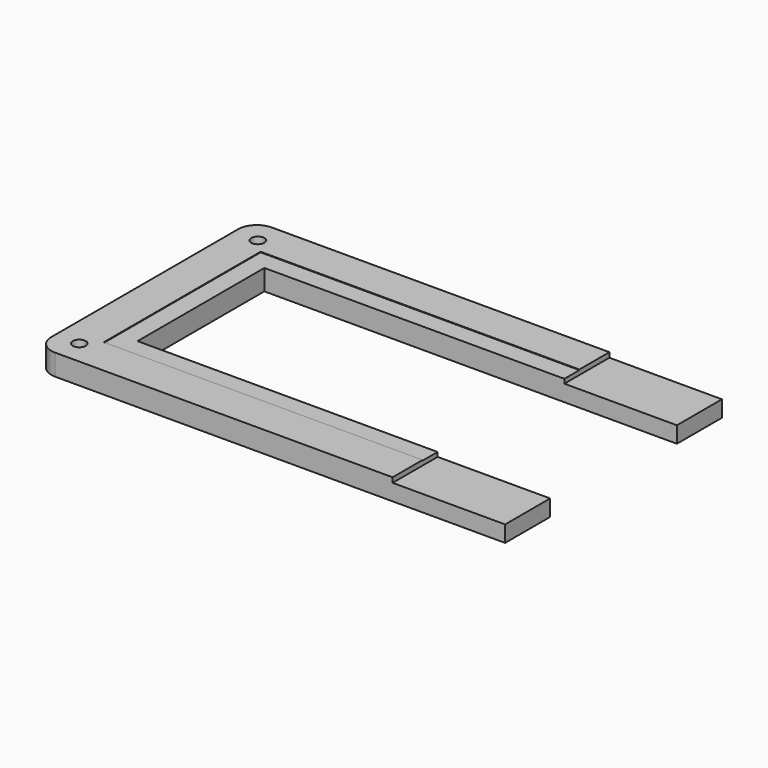
from build123d import *

# Parameters (mm, degrees)
F0_W         = 210
F0_H         = 52.25
F0_W_2       = 200
F0_H_2       = 42.25
F1_DEPTH     = 5.5
F0_W_3       = 230
F0_H_3       = 72.25
F2_DEPTH     = 5.65
F4_DEPTH     = 100
F5_R         = 5
F6_R         = 1.75
F7_DEPTH     = 25
F6_R_2       = 4
F8_DEPTH     = 3
F9_S6_R      = 1.75
F9_T7_DEPTH  = 7
F9_S13_R     = 1.75
F9_T14_DEPTH = 7


# Not quite as in the source:
# - a fillet or chamfer that OpenCascade refuses, or shapes differently, is made with other operations: its cross-section is extruded or revolved along the edge and cut away or added


with BuildPart() as f1:
    # F0 (on Top) → F1 (new body)
    with BuildSketch(Plane.XY):
        with Locations((-28.3456140757, 0)):
            Rectangle(F0_W, F0_H)
        with Locations((-28.3456140757, 0)):
            Rectangle(F0_W_2, F0_H_2, mode=Mode.SUBTRACT)
    extrude(amount=F1_DEPTH)

    # F0 (on Top) → F2 (join)
    with BuildSketch(Plane.XY):
        with Locations((-28.3456140757, 0)):
            Rectangle(F0_W_3, F0_H_3)
        with Locations((-28.3456140757, 0)):
            Rectangle(F0_W, F0_H, mode=Mode.SUBTRACT)
    extrude(amount=F2_DEPTH)

    # F3 (on face) → F4 (cut)
    with BuildSketch(Plane.XZ.offset(36.125)):
        Polygon((-48.3456140757, 5.65), (-48.3456140757, 4.35), (-18.3456140757, 4.35), (-18.3456140757, 0), (86.6543859243, 0), (86.6543859243, 5.65), align=None)
    extrude(amount=-F4_DEPTH, mode=Mode.SUBTRACT)

    # F5
    f5_edges = [f1.edges().sort_by_distance(p)[0] for p in [
        (-143.345614, 36.125, 2.825),
        (-143.345614, -36.125, 2.825),
    ]]
    fillet(f5_edges, radius=F5_R)

    # F6 (on face) → F7 (cut)
    with BuildSketch(Plane.XY):
        with Locations((-136.9816213846, 29.760915786)):
            Circle(F6_R)
        with Locations((-136.9816213846, -29.760915786)):
            Circle(F6_R)
    extrude(amount=F7_DEPTH, mode=Mode.SUBTRACT)

    # F6 (on face) → F8 (cut)
    with BuildSketch(Plane.XY):
        with Locations((-136.9816213846, -29.760915786)):
            Circle(F6_R_2)
        with Locations((-136.9816213846, -29.760915786)):
            Circle(F6_R, mode=Mode.SUBTRACT)
        with Locations((-136.9816213846, 29.760915786)):
            Circle(F6_R_2)
        with Locations((-136.9816213846, 29.760915786)):
            Circle(F6_R, mode=Mode.SUBTRACT)
    extrude(amount=F8_DEPTH, mode=Mode.SUBTRACT)

    # F9: chamfer of 3 x 2.2606621503 on 2 edges, made by hand


with BuildPart() as f9_tool2:
    # F9_s3 → F9_t4 (revolve)
    with BuildSketch(Plane.XZ.offset(-29.760915786)):
        Polygon((-132.9816213846, 0), (-135.2422835349, 3), (-132.9816213846, 3), align=None)
    revolve(axis=Axis((-136.9816213846, 29.760915786, 3), (0, 0, 1)))

    split(bisect_by=Plane.XY, keep=Keep.TOP)

    # F9_s6 → F9_t7 (cut, symmetric)
    with BuildSketch(Plane.XY.offset(1.5)):
        with Locations((-136.9816213846, 29.760915786)):
            Circle(F9_S6_R)
    extrude(amount=F9_T7_DEPTH, both=True, mode=Mode.SUBTRACT)


with BuildPart() as f1_1:
    add(f1.part)

    # F9_t1: union F9_tool2
    add(f9_tool2.part)


with BuildPart() as f9_tool9:
    # F9_s10 → F9_t11 (revolve)
    with BuildSketch(Plane.XZ.offset(29.760915786)):
        Polygon((-132.9816213846, 0), (-135.2422835349, 3), (-132.9816213846, 3), align=None)
    revolve(axis=Axis((-136.9816213846, -29.760915786, 3), (0, 0, 1)))

    split(bisect_by=Plane.XY, keep=Keep.TOP)

    # F9_s13 → F9_t14 (cut, symmetric)
    with BuildSketch(Plane.XY.offset(1.5)):
        with Locations((-136.9816213846, -29.760915786)):
            Circle(F9_S13_R)
    extrude(amount=F9_T14_DEPTH, both=True, mode=Mode.SUBTRACT)


with BuildPart() as f1_2:
    add(f1_1.part)

    # F9_t8: union F9_tool9
    add(f9_tool9.part)


solid = f1_2.part
